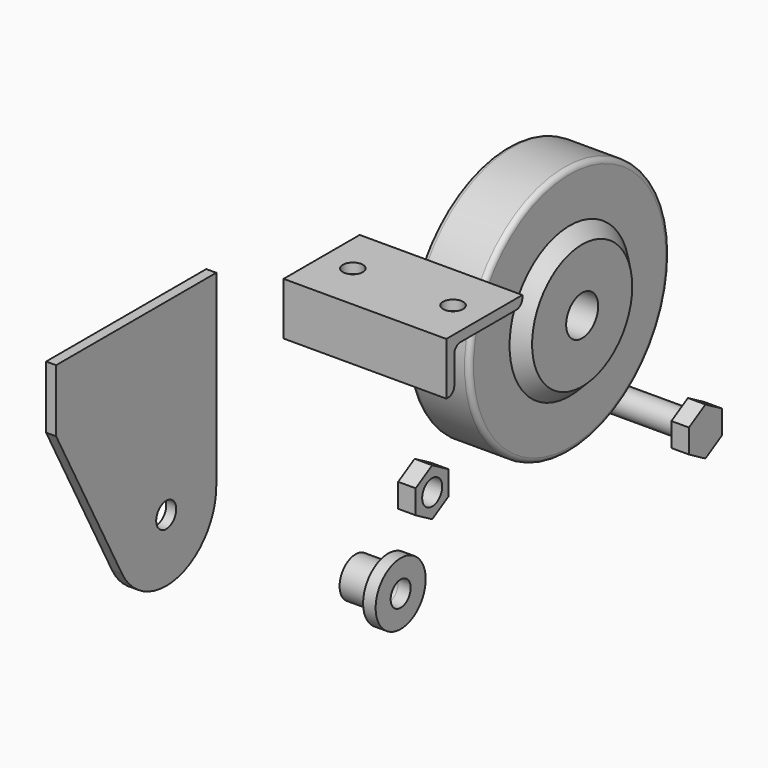
from build123d import *

# Parameters (mm, degrees)
F0_R          = 50
F1_DEPTH      = 12.5
F2_R          = 30
F3_DEPTH      = 5
F3_TAPER      = 45
F4_R          = 2
F5_R          = 8
F6_DEPTH      = 17.5010001
F6_DEPTH_BACK = 17.5010001
F7_R          = 12.5
F7_R_2        = 8
F7_R_3        = 5
F8_DEPTH      = 5
F9_DEPTH      = 13
F10_R         = 5
F11_DEPTH     = 7
F12_DEPTH     = 62
F13_R         = 5
F14_DEPTH     = 7
F15_R         = 5
F16_DEPTH     = 4
F18_DEPTH     = 65
F19_R         = 4
F20_DEPTH     = 25


# Not quite as in the source:
# - a pattern or mirror of a feature is missing from the dataset's text; its kind, count and spacing are read off the source's solid


with BuildPart() as f1:
    # F0 (on Right) → F1 (new body, symmetric)
    with BuildSketch(Plane.YZ):
        Circle(F0_R)
    extrude(amount=F1_DEPTH, both=True)

    # F2 (on face) → F3 (join)
    with BuildSketch(Plane.YZ.offset(12.5)):
        Circle(F2_R)
    f3 = extrude(amount=F3_DEPTH, taper=F3_TAPER)

    # F3_copies: F3 across plane
    add(f3.mirror(Plane(origin=(0, 0, 0), x_dir=(0, 0, -1), z_dir=(-1, 0, 0))))

    # F4
    f4_edges = [f1.edges().sort_by_distance(p)[0] for p in [
        (12.5, -50, 0),
        (-12.5, -50, 0),
    ]]
    fillet(f4_edges, radius=F4_R)

    # F5 (on Right) → F6 (cut, two sides)
    with BuildSketch(Plane.YZ) as f6_sk:
        Circle(F5_R)
    extrude(amount=-F6_DEPTH, mode=Mode.SUBTRACT)
    extrude(f6_sk.sketch, amount=F6_DEPTH_BACK, mode=Mode.SUBTRACT)


with BuildPart() as f8:
    # F7 (on Right) → F8 (new body)
    with BuildSketch(Plane.YZ):
        with Locations((-75.0211775303, -71.3893398643)):
            Circle(F7_R)
        with Locations((-75.0211775303, -71.3893398643)):
            Circle(F7_R_2, mode=Mode.SUBTRACT)
        with Locations((-75.0211775303, -71.3893398643)):
            Circle(F7_R_2)
        with Locations((-75.0211775303, -71.3893398643)):
            Circle(F7_R_3, mode=Mode.SUBTRACT)
    extrude(amount=F8_DEPTH)

    # F7 (on Right) → F9 (join)
    with BuildSketch(Plane.YZ):
        with Locations((-75.0211775303, -71.3893398643)):
            Circle(F7_R_2)
        with Locations((-75.0211775303, -71.3893398643)):
            Circle(F7_R_3, mode=Mode.SUBTRACT)
    extrude(amount=-F9_DEPTH)


with BuildPart() as f11:
    # F10 (on Right) → F11 (new body)
    with BuildSketch(Plane.YZ):
        Polygon((82.9232768221, -69.8334909976), (74.6920183301, -65.0811716914), (66.4607598381, -69.8334909976), (66.4607598381, -79.3381296098), (74.6920183301, -84.090448916), (82.9232768221, -79.3381296098), align=None)
        with Locations((74.6920183301, -74.5858103037)):
            Circle(F10_R, mode=Mode.SUBTRACT)
        with Locations((74.6920183301, -74.5858103037)):
            Circle(F10_R)
    extrude(amount=F11_DEPTH)

    # F10 (on Right) → F12 (join)
    with BuildSketch(Plane.YZ):
        with Locations((74.6920183301, -74.5858103037)):
            Circle(F10_R)
    extrude(amount=-F12_DEPTH)


with BuildPart() as f14:
    # F13 (on Right) → F14 (new body)
    with BuildSketch(Plane.YZ):
        Polygon((-53.5529885899, -35.7310755062), (-61.784247082, -30.9787562001), (-70.015505574, -35.7310755062), (-70.015505574, -45.2357141185), (-61.784247082, -49.9880334246), (-53.5529885899, -45.2357141185), align=None)
        with Locations((-61.784247082, -40.4833948123)):
            Circle(F13_R, mode=Mode.SUBTRACT)
    extrude(amount=F14_DEPTH)


with BuildPart() as f16:
    # F15 (on Right) → F16 (new body)
    with BuildSketch(Plane.YZ):
        with BuildLine():
            Line((-245.8573955297, 53.0606626533), (-212.9162190592, -8.7040432291))
            ThreePointArc((-212.9162190592, -8.7040432291), (-184.7940049038, -21.1928998503), (-165.8573955297, 3.0606626533))
            Line((-165.8573955297, 3.0606626533), (-165.8573955297, 78.0606626533))
            Line((-165.8573955297, 78.0606626533), (-245.8573955297, 78.0606626533))
            Line((-245.8573955297, 78.0606626533), (-245.8573955297, 53.0606626533))
        make_face()
        with Locations((-190.8573955297, 3.0606626533)):
            Circle(F15_R, mode=Mode.SUBTRACT)
    extrude(amount=F16_DEPTH)


with BuildPart() as f18:
    # F17 (on Right) → F18 (new body)
    with BuildSketch(Plane.YZ):
        with BuildLine():
            Line((-89.2400319576, 57.9238541722), (-89.2400319576, 58.9238541722))
            Line((-89.2400319576, 58.9238541722), (-127.2400319576, 58.9238541722))
            Line((-127.2400319576, 58.9238541722), (-127.2400319576, 37.9238541722))
            Line((-127.2400319576, 37.9238541722), (-126.2400319576, 37.9238541722))
            ThreePointArc((-126.2400319576, 37.9238541722), (-124.1187116141, 38.8025338287), (-123.2400319576, 40.9238541722))
            Line((-123.2400319576, 40.9238541722), (-123.2400319576, 51.9238541722))
            ThreePointArc((-123.2400319576, 51.9238541722), (-122.3613523012, 54.0451745158), (-120.2400319576, 54.9238541722))
            Line((-120.2400319576, 54.9238541722), (-92.2400319576, 54.9238541722))
            ThreePointArc((-92.2400319576, 54.9238541722), (-90.1187116141, 55.8025338287), (-89.2400319576, 57.9238541722))
        make_face()
    extrude(amount=F18_DEPTH)

    # F19 (on face) → F20 (cut)
    with BuildSketch(Plane.XY.offset(58.9238541722)):
        with Locations((52.5, -108.2400319576)):
            Circle(F19_R)
        with Locations((12.5, -108.2400319576)):
            Circle(F19_R)
    extrude(amount=-F20_DEPTH, mode=Mode.SUBTRACT)


solid = Compound([f1.part, f8.part, f11.part, f14.part, f16.part, f18.part])
